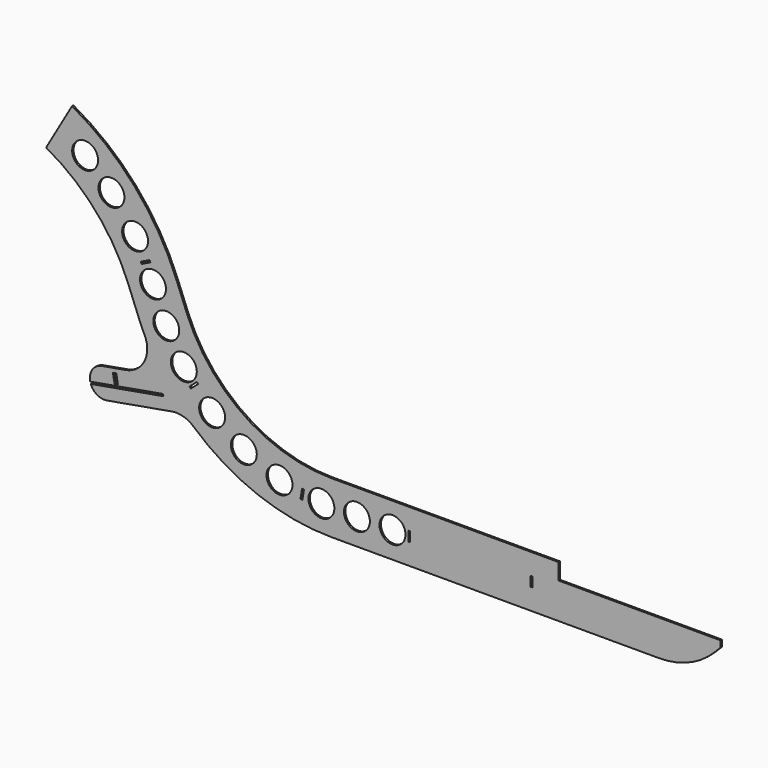
from build123d import *

# Parameters (mm, degrees)
F0_R     = 25.4
F0_W     = 3.81
F0_H     = 19.05
F1_DEPTH = 3.429


# Not quite as in the source:
# - ends of sketch curves that miss each other by under 0.0002 mm in the source are joined


with BuildPart() as f1:
    # F0 (on Front) → F1 (new body)
    with BuildSketch(Plane.XZ):
        with BuildLine():
            ThreePointArc((-642.1692497265, -473.1768646252), (-619.4825639758, -474.3339275445), (-599.5683960075, -485.2632650852))
            ThreePointArc((-599.5683960075, -485.2632650852), (-473.9081608396, -561.5426017902), (-329.3321582, -588.1285164))
            Line((-329.3321582, -588.1285164), (312.391679, -588.1285164))
            ThreePointArc((312.391679, -588.1285164), (370.7126340924, -576.5277571547), (420.1547524528, -543.4915898528))
            Line((420.1547524528, -543.4915898528), (432.6678418, -530.9785164))
            Line((432.6678418, -530.9785164), (432.6678418, -518.2785164))
            Line((432.6678418, -518.2785164), (115.1678418, -518.2785164))
            Line((115.1678418, -518.2785164), (115.1678418, -486.5285164))
            Line((115.1678418, -486.5285164), (-329.3321582, -486.5285164))
            ThreePointArc((-329.3321582, -486.5285164), (-500.4183293998, -433.9834708096), (-612.5167665735, -294.4650126217))
            Line((-612.5167665735, -294.4650126217), (-633.7122454, -241.2238))
            ThreePointArc((-633.7122454, -241.2238), (-715.4828245955, -108.0397407431), (-837.3321571082, -10.1767620246))
            Line((-837.3321571082, -10.1767620246), (-888.1321582, -98.1649548))
            ThreePointArc((-888.1321582, -98.1649548), (-792.2711581527, -174.5413586603), (-728.0333576386, -278.9261845185))
            Line((-728.0333576386, -278.9261845185), (-706.971662, -331.8929862))
            ThreePointArc((-706.971662, -331.8929862), (-701.288086285, -345.465340488), (-695.1169115223, -358.8230511462))
            ThreePointArc((-695.1169115223, -358.8230511462), (-695.6103607346, -404.0881567784), (-732.0186808394, -430.9880994311))
            Line((-732.0186808394, -430.9880994311), (-778.7941498, -439.2359008))
            ThreePointArc((-778.7941498, -439.2359008), (-797.5979576606, -451.5111596623), (-801.724697479, -473.5845717908))
            Line((-801.724697479, -473.5845717908), (-659.172037, -448.448684))
            Line((-659.172037, -448.448684), (-658.5104432, -452.2007974))
            Line((-658.5104432, -452.2007974), (-800.6426456, -477.2625456))
            ThreePointArc((-800.6426456, -477.2625456), (-788.0677244467, -492.1533513081), (-768.8701676538, -495.5176466233))
            Line((-768.8701676538, -495.5176466233), (-642.1692497265, -473.1768646252))
        make_face()
        Polygon((-753.9383956, -462.4504086), (-757.24639, -443.6898162), (-750.74272, -442.543057), (-747.4347256, -461.3036494), align=None, mode=Mode.SUBTRACT)
        with Locations((-562.9950386, -449.5436526)):
            Circle(F0_R, mode=Mode.SUBTRACT)
        with Locations((-431.0197374, -522.7745704)):
            Circle(F0_R, mode=Mode.SUBTRACT)
        with Locations((-349.0011308, -536.6188658)):
            Circle(F0_R, mode=Mode.SUBTRACT)
        Polygon((-383.0809204, -523.6095192), (-386.1430682, -542.411793), (-389.9035128, -541.7993482), (-386.841365, -522.9970744), align=None, mode=Mode.SUBTRACT)
        with Locations((-279.3916688, -536.6188658)):
            Circle(F0_R, mode=Mode.SUBTRACT)
        with Locations((-500.8834026, -493.095026)):
            Circle(F0_R, mode=Mode.SUBTRACT)
        Polygon((-590.2629546, -409.075509), (-604.6945742, -421.510587), (-607.1815898, -418.624258), (-592.7499702, -406.1892054), align=None, mode=Mode.SUBTRACT)
        with Locations((-618.3772494, -388.5352402)):
            Circle(F0_R, mode=Mode.SUBTRACT)
        with Locations((-652.7354484, -328.9401854)):
            Circle(F0_R, mode=Mode.SUBTRACT)
        with Locations((-209.7308988, -536.6188658)):
            Circle(F0_R, mode=Mode.SUBTRACT)
        with Locations((-176.9321582, -537.3285164)):
            Rectangle(F0_W, F0_H, mode=Mode.SUBTRACT)
        with Locations((62.7803418, -537.3285164)):
            Rectangle(F0_W, F0_H, mode=Mode.SUBTRACT)
        with Locations((-678.731434, -265.7196362)):
            Circle(F0_R, mode=Mode.SUBTRACT)
        Polygon((-683.8231434, -229.7111992), (-700.9451564, -238.0621858), (-702.6153588, -234.6377832), (-685.4933458, -226.2867966), align=None, mode=Mode.SUBTRACT)
        with Locations((-713.8615898, -194.4801292)):
            Circle(F0_R, mode=Mode.SUBTRACT)
        with Locations((-760.120654, -134.1457058)):
            Circle(F0_R, mode=Mode.SUBTRACT)
        with Locations((-811.7017548, -87.0353098)):
            Circle(F0_R, mode=Mode.SUBTRACT)
    extrude(amount=F1_DEPTH)


solid = f1.part
